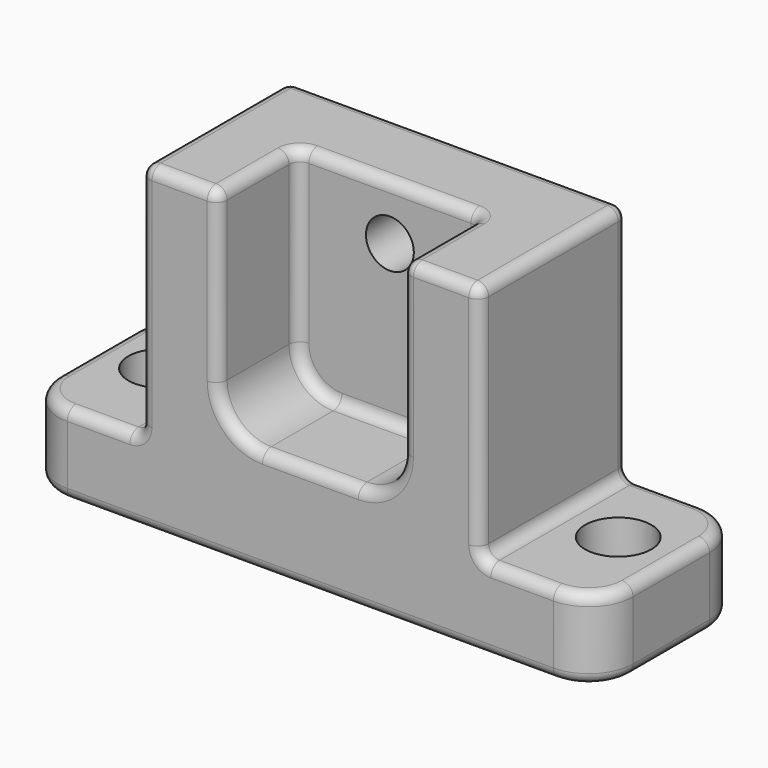
from build123d import *

# Parameters (mm, degrees)
F1_DEPTH = 25
F3_DEPTH = 27
F4_R     = 6.5
F5_DEPTH = 25
F6_R     = 6.5
F7_DEPTH = 22.001
F8_R     = 9
F8_R_2   = 6.5
F9_DEPTH = 10
F10_R    = 12
F11_R    = 3


# Not quite as in the source:
# - a pattern or mirror of a feature is missing from the dataset's text; its kind, count and spacing are read off the source's solid


with BuildPart() as f1:
    # F0 (on Front) → F1 (new body, symmetric)
    with BuildSketch(Plane.XZ):
        Polygon((46, 87), (0, 87), (-46, 87), (-46, 22), (-78, 22), (-78, 0), (0, 0), (78, 0), (78, 22), (46, 22), align=None)
    extrude(amount=F1_DEPTH, both=True)

    # F2 (on face) → F3 (cut)
    with BuildSketch(Plane.XZ.offset(25)):
        Polygon((25, 87), (0, 87), (-25, 87), (-25, 29), (0, 29), (25, 29), align=None)
    extrude(amount=-F3_DEPTH, mode=Mode.SUBTRACT)

    # F4 (on face) → F5 (cut)
    with BuildSketch(Plane.XZ.offset(-2)):
        with Locations((0, 72)):
            Circle(F4_R)
    extrude(amount=-F5_DEPTH, mode=Mode.SUBTRACT)

    # F6 (on face) → F7 (cut, through all)
    with BuildSketch(Plane.XY.offset(22)):
        with Locations((62, 2)):
            Circle(F6_R)
    f7 = extrude(amount=-F7_DEPTH, mode=Mode.SUBTRACT)

    # F7_copies: F7 across plane
    add(f7.mirror(Plane(origin=(0, 0, 0), x_dir=(0, 0, -1), z_dir=(-1, 0, 0))), mode=Mode.SUBTRACT)

    # F8 (on face) → F9 (cut)
    with BuildSketch(Plane.XY.offset(22)):
        with Locations((62, 2)):
            Circle(F8_R)
        with Locations((62, 2)):
            Circle(F8_R_2, mode=Mode.SUBTRACT)
    f9 = extrude(amount=-F9_DEPTH, mode=Mode.SUBTRACT)

    # F9_copies: F9 across plane
    add(f9.mirror(Plane(origin=(0, 0, 0), x_dir=(0, 0, -1), z_dir=(-1, 0, 0))), mode=Mode.SUBTRACT)

    # F10
    f10_edges = [f1.edges().sort_by_distance(p)[0] for p in [
        (-25, -11.5, 29),
        (25, -11.5, 29),
        (78, -25, 11),
        (-78, -25, 11),
        (-78, 25, 11),
        (78, 25, 11),
    ]]
    fillet(f10_edges, radius=F10_R)

    # F11
    f11_edges = [f1.edges().sort_by_distance(p)[0] for p in [
        (46, 0, 87),
        (35.5, -25, 87),
        (25, -11.5, 87),
        (0, 2, 87),
        (-25, -11.5, 87),
        (-35.5, -25, 87),
        (-46, 0, 87),
        (0, 25, 87),
        (-25, -25, 64),
        (-21.485281, -25, 32.514719),
        (0, -25, 29),
        (-46, -25, 54.5),
        (21.485281, -25, 32.514719),
        (-56, -25, 22),
        (25, -25, 64),
        (-66, -25, 11),
        (0, -25, 0),
        (46, -25, 54.5),
        (66, -25, 11),
        (56, -25, 22),
        (46, 25, 54.5),
        (46, 0, 22),
        (-46, 25, 54.5),
        (-46, 0, 22),
        (-25, 2, 64),
        (-21.485281, 2, 32.514719),
        (0, 2, 29),
        (21.485281, 2, 32.514719),
        (-56, 25, 22),
        (-74.485281, 21.485281, 22),
        (-78, 0, 22),
        (-74.485281, -21.485281, 22),
        (25, 2, 64),
        (-74.485281, -21.485281, 0),
        (-78, 0, 0),
        (-74.485281, 21.485281, 0),
        (0, 25, 0),
        (74.485281, 21.485281, 0),
        (74.485281, -21.485281, 0),
        (78, 0, 0),
        (74.485281, -21.485281, 22),
        (56, 25, 22),
        (74.485281, 21.485281, 22),
        (78, 0, 22),
    ]]
    fillet(f11_edges, radius=F11_R)


solid = f1.part
